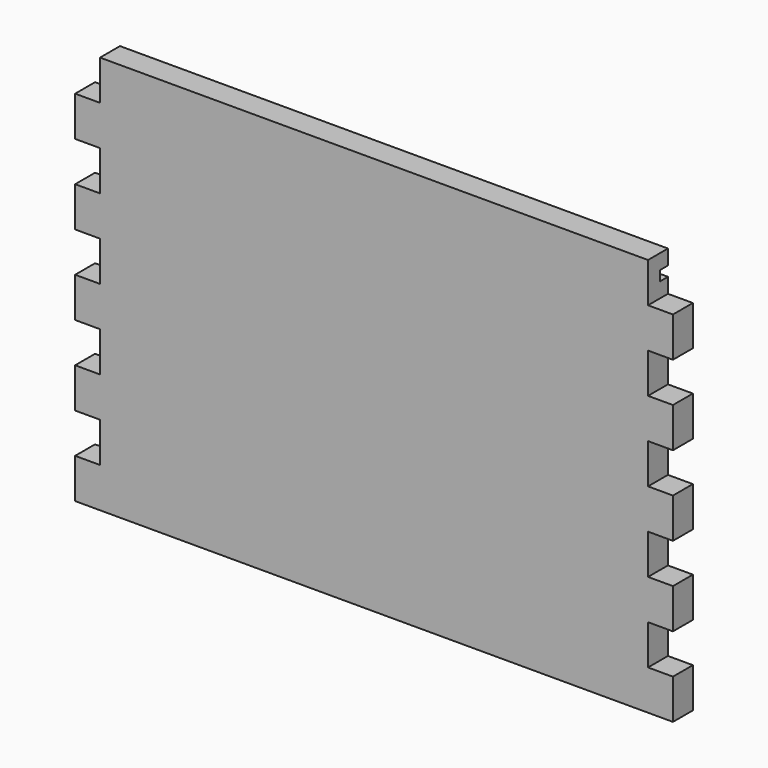
from build123d import *

# Parameters (mm, degrees)
F2_DEPTH = 5
F3_W     = 2
F3_H     = 2
F4_DEPTH = 120.001


# Not quite as in the source:
# - a feature names something its author has since deleted; it is built from what else it names


with BuildPart() as f2:
    # F1 (on Front) → F2 (new body)
    with BuildSketch(Plane.XZ):
        Polygon((55, -8), (55, 0), (-55, 0), (-55, -8), (-60, -8), (-60, -16), (-55, -16), (-55, -24), (-60, -24), (-60, -32), (-55, -32), (-55, -40), (-60, -40), (-60, -48), (-55, -48), (-55, -56), (-60, -56), (-60, -64), (-55, -64), (-55, -72), (-60, -72), (-60, -80), (60, -80), (60, -72), (55, -72), (55, -64), (60, -64), (60, -56), (55, -56), (55, -48), (60, -48), (60, -40), (55, -40), (55, -32), (60, -32), (60, -24), (55, -24), (55, -16), (60, -16), (60, -8), align=None)
    extrude(amount=F2_DEPTH)

    # F3 (on face) → F4 (cut, through all)
    with BuildSketch(Plane.YZ.offset(60)):
        with Locations((-1, -4)):
            Rectangle(F3_W, F3_H)
    extrude(amount=-F4_DEPTH, mode=Mode.SUBTRACT)


solid = f2.part
